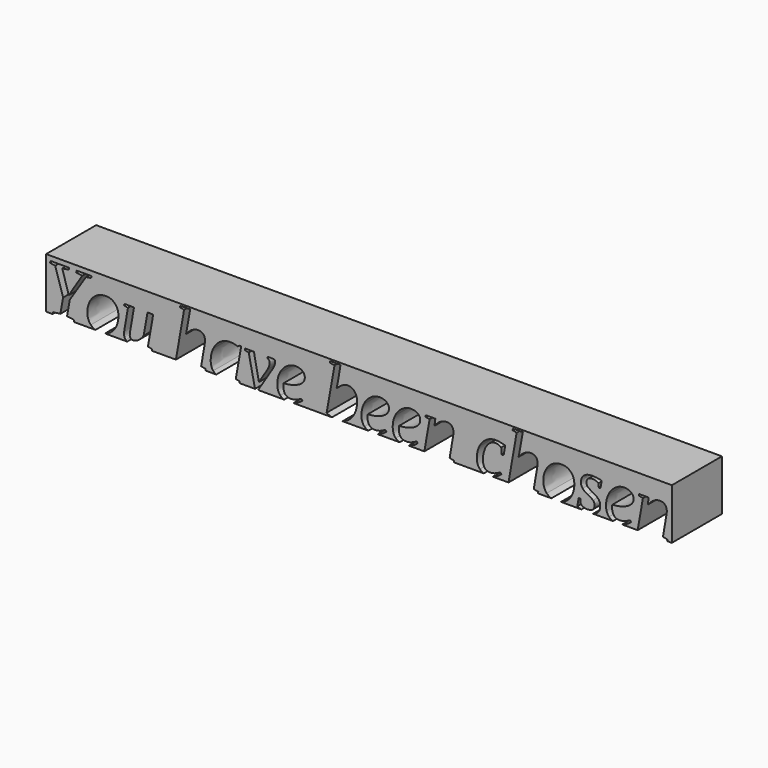
from build123d import *

# Parameters (mm, degrees)
F1_DEPTH = 6.35


with BuildPart() as f1:
    # F0 (on Front) → F1 (new body)
    with BuildSketch(Plane.XZ):
        with BuildLine():
            Line((-250.0064443607, 5.1488298434), (-313.5064443607, 5.1488298434))
            Line((-313.5064443607, 5.1488298434), (-313.5064443607, 0))
            Line((-313.5064443607, 0), (-312.8460801164, 0))
            Line((-312.8460801164, 0), (-312.8114417212, 0.1854830195))
            Line((-312.8114417212, 0.1854830195), (-312.0538664969, 0.2793418969))
            Line((-312.0538664969, 0.2793418969), (-311.7812288055, 1.8224265353))
            Line((-311.7812288055, 1.8224265353), (-312.584616101, 4.4068977653))
            Line((-312.584616101, 4.4068977653), (-313.0974878236, 4.4974045399))
            Line((-313.0974878236, 4.4974045399), (-313.0628494284, 4.6828875594))
            Line((-313.0628494284, 4.6828875594), (-311.1532682213, 4.6828875594))
            Line((-311.1532682213, 4.6828875594), (-311.1879066165, 4.4974045399))
            Line((-311.1879066165, 4.4974045399), (-311.8650313746, 4.4068977653))
            Line((-311.8650313746, 4.4068977653), (-311.2091366007, 2.2168572937))
            Line((-311.2091366007, 2.2168572937), (-309.8370092032, 4.4068977653))
            Line((-309.8370092032, 4.4068977653), (-310.4515613763, 4.4974045399))
            Line((-310.4515613763, 4.4974045399), (-310.4158056135, 4.6828875594))
            Line((-310.4158056135, 4.6828875594), (-308.8939509593, 4.6828875594))
            Line((-308.8939509593, 4.6828875594), (-308.9285893545, 4.4974045399))
            Line((-308.9285893545, 4.4974045399), (-309.4559868558, 4.4068977653))
            Line((-309.4559868558, 4.4068977653), (-311.1041040475, 1.8436565194))
            Line((-311.1041040475, 1.8436565194), (-311.3800938416, 0.2793418969))
            Line((-311.3800938416, 0.2793418969), (-310.6504528069, 0.1854830195))
            Line((-310.6504528069, 0.1854830195), (-310.6850912021, 0))
            Line((-310.6850912021, 0), (-308.4992285411, 0))
            add(Edge.make_bspline(
                [(-308.4992285411, 0), (-308.7698389481, 0.0914468075), (-308.9671385363, 0.3016892486)],
                knots=[0.4349588362, 0.4349588362, 0.4349588362, 1, 1, 1], degree=2))
            add(Edge.make_bspline(
                [(-308.9671385363, 0.3016892486), (-309.3163159074, 0.6737726553), (-309.3163159074, 1.3062027098)],
                knots=[0, 0, 0, 1, 1, 1], degree=2))
            add(Edge.make_bspline(
                [(-309.3163159074, 1.3062027098), (-309.3163159074, 1.8682386064), (-309.0755231923, 2.3464719338)],
                knots=[0, 0, 0, 1, 1, 1], degree=2))
            add(Edge.make_bspline(
                [(-309.0755231923, 2.3464719338), (-308.8347304772, 2.8247052613), (-308.4067786911, 3.0973429527)],
                knots=[0, 0, 0, 1, 1, 1], degree=2))
            add(Edge.make_bspline(
                [(-308.4067786911, 3.0973429527), (-307.9788269051, 3.369980644), (-307.4447251983, 3.369980644)],
                knots=[0, 0, 0, 1, 1, 1], degree=2))
            add(Edge.make_bspline(
                [(-307.4447251983, 3.369980644), (-306.8659287879, 3.369980644), (-306.5167514168, 2.9978972374)],
                knots=[0, 0, 0, 1, 1, 1], degree=2))
            add(Edge.make_bspline(
                [(-306.5167514168, 2.9978972374), (-306.1675740457, 2.6258138307), (-306.1675740457, 1.9933837762)],
                knots=[0, 0, 0, 1, 1, 1], degree=2))
            add(Edge.make_bspline(
                [(-306.1675740457, 1.9933837762), (-306.1675740457, 1.4313478796), (-306.4083667608, 0.9531145522)],
                knots=[0, 0, 0, 1, 1, 1], degree=2))
            add(Edge.make_bspline(
                [(-306.4083667608, 0.9531145522), (-306.6491594759, 0.4748812247), (-307.0765525782, 0.2022435333)],
                knots=[0, 0, 0, 1, 1, 1], degree=2))
            add(Edge.make_bspline(
                [(-307.0765525782, 0.2022435333), (-307.2867741608, 0.0681413996), (-307.523082673, 0)],
                knots=[0, 0, 0, 0.4918693856, 0.4918693856, 0.4918693856], degree=2))
            Line((-307.523082673, 0), (-305.2797553892, 0))
            add(Edge.make_bspline(
                [(-305.2797553892, 0), (-305.3594784168, 0.0425514012), (-305.4194964458, 0.1067086046)],
                knots=[0.6632365324, 0.6632365324, 0.6632365324, 1, 1, 1], degree=2))
            add(Edge.make_bspline(
                [(-305.4194964458, 0.1067086046), (-305.5977165761, 0.2972197783), (-305.5977165761, 0.6525426711)],
                knots=[0, 0, 0, 1, 1, 1], degree=2))
            add(Edge.make_bspline(
                [(-305.5977165761, 0.6525426711), (-305.5977165761, 0.7050589477), (-305.5787213271, 0.839701742)],
                knots=[0, 0, 0, 1, 1, 1], degree=2))
            add(Edge.make_bspline(
                [(-305.5787213271, 0.839701742), (-305.5597260781, 0.9743445363), (-305.2032858177, 3.0414745733)],
                knots=[0, 0, 0, 1, 1, 1], degree=2))
            Line((-305.2032858177, 3.0414745733), (-305.5910123705, 3.1252771424))
            Line((-305.5910123705, 3.1252771424), (-305.5630781808, 3.2828259722))
            Line((-305.5630781808, 3.2828259722), (-304.582029439, 3.2828259722))
            Line((-304.582029439, 3.2828259722), (-304.9384696994, 1.2536864332))
            add(Edge.make_bspline(
                [(-304.9384696994, 1.2536864332), (-305.0178027981, 0.8134436037), (-305.0178027981, 0.6737726553)],
                knots=[0, 0, 0, 1, 1, 1], degree=2))
            add(Edge.make_bspline(
                [(-305.0178027981, 0.6737726553), (-305.0178027981, 0.517341193), (-304.9340002291, 0.4195715291)],
                knots=[0, 0, 0, 1, 1, 1], degree=2))
            add(Edge.make_bspline(
                [(-304.9340002291, 0.4195715291), (-304.85019766, 0.3218018652), (-304.6691841108, 0.3218018652)],
                knots=[0, 0, 0, 1, 1, 1], degree=2))
            add(Edge.make_bspline(
                [(-304.6691841108, 0.3218018652), (-304.4077200953, 0.3218018652), (-304.1037961115, 0.5396885448)],
                knots=[0, 0, 0, 1, 1, 1], degree=2))
            add(Edge.make_bspline(
                [(-304.1037961115, 0.5396885448), (-303.7998721277, 0.7575752244), (-303.6043327999, 1.0760249868)],
                knots=[0, 0, 0, 1, 1, 1], degree=2))
            Line((-303.6043327999, 1.0760249868), (-303.216606247, 3.2828259722))
            Line((-303.216606247, 3.2828259722), (-302.6366924691, 3.2828259722))
            Line((-302.6366924691, 3.2828259722), (-303.1707941759, 0.2447035017))
            Line((-303.1707941759, 0.2447035017), (-302.7596029037, 0.1575488298))
            Line((-302.7596029037, 0.1575488298), (-302.7875370934, 0))
            Line((-302.7875370934, 0), (-300.3326805036, 0))
            Line((-300.3326805036, 0), (-299.5047111212, 4.7208780574))
            Line((-299.5047111212, 4.7208780574), (-299.917019761, 4.8046806264))
            Line((-299.917019761, 4.8046806264), (-299.8890855713, 4.9622294563))
            Line((-299.8890855713, 4.9622294563), (-298.8834547425, 4.9622294563))
            Line((-298.8834547425, 4.9622294563), (-299.253303414, 2.8805736407))
            Line((-299.253303414, 2.8805736407), (-299.3091717934, 2.6157575224))
            add(Edge.make_bspline(
                [(-299.3091717934, 2.6157575224), (-299.0298298965, 2.9822540911), (-298.7102627664, 3.1761173676)],
                knots=[0, 0, 0, 1, 1, 1], degree=2))
            add(Edge.make_bspline(
                [(-298.7102627664, 3.1761173676), (-298.3906956364, 3.369980644), (-298.0834195498, 3.369980644)],
                knots=[0, 0, 0, 1, 1, 1], degree=2))
            add(Edge.make_bspline(
                [(-298.0834195498, 3.369980644), (-297.7314487598, 3.369980644), (-297.5532286295, 3.1794694704)],
                knots=[0, 0, 0, 1, 1, 1], degree=2))
            add(Edge.make_bspline(
                [(-297.5532286295, 3.1794694704), (-297.3750084993, 2.9889582967), (-297.3750084993, 2.6325180362)],
                knots=[0, 0, 0, 1, 1, 1], degree=2))
            add(Edge.make_bspline(
                [(-297.3750084993, 2.6325180362), (-297.3750084993, 2.58447123), (-297.3889755942, 2.4827907795)],
                knots=[0, 0, 0, 1, 1, 1], degree=2))
            add(Edge.make_bspline(
                [(-297.3889755942, 2.4827907795), (-297.402942689, 2.3811103291), (-297.7694392577, 0.2413513989)],
                knots=[0, 0, 0, 1, 1, 1], degree=2))
            Line((-297.7694392577, 0.2413513989), (-297.3124359144, 0.1575488298))
            Line((-297.3124359144, 0.1575488298), (-297.3403701041, 0))
            Line((-297.3403701041, 0), (-296.2384625881, 0))
            add(Edge.make_bspline(
                [(-296.2384625881, 0), (-296.4137627106, 0.0777425781), (-296.5453630656, 0.2374406124)],
                knots=[0.4868098623, 0.4868098623, 0.4868098623, 1, 1, 1], degree=2))
            add(Edge.make_bspline(
                [(-296.5453630656, 0.2374406124), (-296.8017989269, 0.5486274855), (-296.8017989269, 1.0927855006)],
                knots=[0, 0, 0, 1, 1, 1], degree=2))
            add(Edge.make_bspline(
                [(-296.8017989269, 1.0927855006), (-296.8017989269, 1.703985571), (-296.5347480735, 2.2364112265)],
                knots=[0, 0, 0, 1, 1, 1], degree=2))
            add(Edge.make_bspline(
                [(-296.5347480735, 2.2364112265), (-296.2676972201, 2.7688368819), (-295.8207501851, 3.0677327116)],
                knots=[0, 0, 0, 1, 1, 1], degree=2))
            add(Edge.make_bspline(
                [(-295.8207501851, 3.0677327116), (-295.37380315, 3.3666285413), (-294.8497577515, 3.3666285413)],
                knots=[0, 0, 0, 1, 1, 1], degree=2))
            add(Edge.make_bspline(
                [(-294.8497577515, 3.3666285413), (-294.4273928034, 3.3666285413), (-294.0541920292, 3.2191360197)],
                knots=[0, 0, 0, 1, 1, 1], degree=2))
            Line((-294.0541920292, 3.2191360197), (-293.8966431993, 3.3386943516))
            Line((-293.8966431993, 3.3386943516), (-293.7089254446, 3.3386943516))
            Line((-293.7089254446, 3.3386943516), (-294.2597876653, 0.2447035017))
            Line((-294.2597876653, 0.2447035017), (-293.8653569069, 0.1575488298))
            Line((-293.8653569069, 0.1575488298), (-293.8932910966, 0))
            Line((-293.8932910966, 0), (-292.3025629003, 0))
            Line((-292.3025629003, 0), (-292.9468807499, 3.0381224705))
            Line((-292.9468807499, 3.0381224705), (-293.3413115083, 3.1252771424))
            Line((-293.3413115083, 3.1252771424), (-293.3100252159, 3.2828259722))
            Line((-293.3100252159, 3.2828259722), (-292.4161311458, 3.2828259722))
            Line((-292.4161311458, 3.2828259722), (-291.9099636287, 0.7262889319))
            Line((-291.9099636287, 0.7262889319), (-291.0406516456, 2.1442284005))
            add(Edge.make_bspline(
                [(-291.0406516456, 2.1442284005), (-290.8171781281, 2.5073728664), (-290.8171781281, 2.8180010558)],
                knots=[0, 0, 0, 1, 1, 1], degree=2))
            add(Edge.make_bspline(
                [(-290.8171781281, 2.8180010558), (-290.8171781281, 2.9476156959), (-290.890365705, 3.0241553757)],
                knots=[0, 0, 0, 1, 1, 1], degree=2))
            add(Edge.make_bspline(
                [(-290.890365705, 3.0241553757), (-290.963553282, 3.1006950554), (-291.0473558511, 3.1252771424)],
                knots=[0, 0, 0, 1, 1, 1], degree=2))
            Line((-291.0473558511, 3.1252771424), (-291.0194216614, 3.2828259722))
            Line((-291.0194216614, 3.2828259722), (-290.356822682, 3.2828259722))
            add(Edge.make_bspline(
                [(-290.356822682, 3.2828259722), (-290.2651985398, 3.2023755059), (-290.2651985398, 3.0627045575)],
                knots=[0, 0, 0, 1, 1, 1], degree=2))
            add(Edge.make_bspline(
                [(-290.2651985398, 3.0627045575), (-290.2651985398, 2.7554284709), (-290.5557141126, 2.2939556572)],
                knots=[0, 0, 0, 1, 1, 1], degree=2))
            Line((-290.5557141126, 2.2939556572), (-291.9888943483, 0))
            Line((-291.9888943483, 0), (-289.3441800038, 0))
            add(Edge.make_bspline(
                [(-289.3441800038, 0), (-289.5780654992, 0.0788026603), (-289.7394770899, 0.2458208693)],
                knots=[0.4718207721, 0.4718207721, 0.4718207721, 1, 1, 1], degree=2))
            add(Edge.make_bspline(
                [(-289.7394770899, 0.2458208693), (-290.0450771251, 0.5620358965), (-290.0450771251, 1.1520059828)],
                knots=[0, 0, 0, 1, 1, 1], degree=2))
            add(Edge.make_bspline(
                [(-290.0450771251, 1.1520059828), (-290.0450771251, 1.7352718635), (-289.798697572, 2.2397633292)],
                knots=[0, 0, 0, 1, 1, 1], degree=2))
            add(Edge.make_bspline(
                [(-289.798697572, 2.2397633292), (-289.552318019, 2.744254795), (-289.115985976, 3.0571177195)],
                knots=[0, 0, 0, 1, 1, 1], degree=2))
            add(Edge.make_bspline(
                [(-289.115985976, 3.0571177195), (-288.6796539331, 3.369980644), (-288.2014206056, 3.369980644)],
                knots=[0, 0, 0, 1, 1, 1], degree=2))
            add(Edge.make_bspline(
                [(-288.2014206056, 3.369980644), (-287.772351452, 3.369980644), (-287.5120048041, 3.1727652648)],
                knots=[0, 0, 0, 1, 1, 1], degree=2))
            add(Edge.make_bspline(
                [(-287.5120048041, 3.1727652648), (-287.2516581562, 2.9755498856), (-287.2516581562, 2.6537480204)],
                knots=[0, 0, 0, 1, 1, 1], degree=2))
            add(Edge.make_bspline(
                [(-287.2516581562, 2.6537480204), (-287.2516581562, 2.1788667957), (-287.8382761397, 1.8436565194)],
                knots=[0, 0, 0, 1, 1, 1], degree=2))
            add(Edge.make_bspline(
                [(-287.8382761397, 1.8436565194), (-288.4248941231, 1.5084462432), (-289.4126470705, 1.4425215555)],
                knots=[0, 0, 0, 1, 1, 1], degree=2))
            Line((-289.4126470705, 1.4425215555), (-289.4271728492, 1.1877617456))
            add(Edge.make_bspline(
                [(-289.4271728492, 1.1877617456), (-289.4271728492, 0.7441668133), (-289.240572462, 0.5190172444)],
                knots=[0, 0, 0, 1, 1, 1], degree=2))
            add(Edge.make_bspline(
                [(-289.240572462, 0.5190172444), (-289.0539720749, 0.2938676755), (-288.6863581386, 0.2938676755)],
                knots=[0, 0, 0, 1, 1, 1], degree=2))
            add(Edge.make_bspline(
                [(-288.6863581386, 0.2938676755), (-288.3723778465, 0.2938676755), (-288.1070030445, 0.4000175963)],
                knots=[0, 0, 0, 1, 1, 1], degree=2))
            add(Edge.make_bspline(
                [(-288.1070030445, 0.4000175963), (-287.8416282424, 0.5061675172), (-287.6114505194, 0.6424863628)],
                knots=[0, 0, 0, 1, 1, 1], degree=2))
            Line((-287.6114505194, 0.6424863628), (-287.5097700689, 0.4961112089))
            add(Edge.make_bspline(
                [(-287.5097700689, 0.4961112089), (-287.8315719341, 0.2234735175), (-288.1891295622, 0.0765396797)],
                knots=[0, 0, 0, 1, 1, 1], degree=2))
            add(Edge.make_bspline(
                [(-288.1891295622, 0.0765396797), (-288.2991995892, 0.031307778), (-288.4058812363, 0)],
                knots=[0, 0, 0, 0.3078385647, 0.3078385647, 0.3078385647], degree=2))
            Line((-288.4058812363, 0), (-284.4901280472, 0))
            add(Edge.make_bspline(
                [(-284.4901280472, 0), (-284.5063254791, 0.0040723352), (-284.5224878236, 0.0083802569)],
                knots=[0.9453131869, 0.9453131869, 0.9453131869, 1, 1, 1], degree=2))
            add(Edge.make_bspline(
                [(-284.5224878236, 0.0083802569), (-284.8180315505, 0.0871546718), (-285.0370355977, 0.2234735175)],
                knots=[0, 0, 0, 1, 1, 1], degree=2))
            Line((-285.0370355977, 0.2234735175), (-284.2381177726, 4.7208780574))
            Line((-284.2381177726, 4.7208780574), (-284.7018253214, 4.8046806264))
            Line((-284.7018253214, 4.8046806264), (-284.6738911317, 4.9622294563))
            Line((-284.6738911317, 4.9622294563), (-283.6269177022, 4.9622294563))
            Line((-283.6269177022, 4.9622294563), (-283.8850296149, 3.4224969206))
            add(Edge.make_bspline(
                [(-283.8850296149, 3.4224969206), (-283.9442500971, 3.0235966919), (-284.0213484606, 2.7476068978)],
                knots=[0, 0, 0, 1, 1, 1], degree=2))
            add(Edge.make_bspline(
                [(-284.0213484606, 2.7476068978), (-283.7420065637, 3.0347703678), (-283.4470215206, 3.2023755059)],
                knots=[0, 0, 0, 1, 1, 1], degree=2))
            add(Edge.make_bspline(
                [(-283.4470215206, 3.2023755059), (-283.1520364775, 3.369980644), (-282.9039808731, 3.369980644)],
                knots=[0, 0, 0, 1, 1, 1], degree=2))
            add(Edge.make_bspline(
                [(-282.9039808731, 3.369980644), (-282.4670901464, 3.369980644), (-282.2056261309, 3.0571177195)],
                knots=[0, 0, 0, 1, 1, 1], degree=2))
            add(Edge.make_bspline(
                [(-282.2056261309, 3.0571177195), (-281.9441621154, 2.744254795), (-281.9441621154, 2.2034488826)],
                knots=[0, 0, 0, 1, 1, 1], degree=2))
            add(Edge.make_bspline(
                [(-281.9441621154, 2.2034488826), (-281.9441621154, 1.6023051205), (-282.2039500795, 1.0698794651)],
                knots=[0, 0, 0, 1, 1, 1], degree=2))
            add(Edge.make_bspline(
                [(-282.2039500795, 1.0698794651), (-282.4637380436, 0.5374538096), (-282.9213000707, 0.2335298258)],
                knots=[0, 0, 0, 1, 1, 1], degree=2))
            add(Edge.make_bspline(
                [(-282.9213000707, 0.2335298258), (-283.158652726, 0.075874338), (-283.4184049976, 0)],
                knots=[0, 0, 0, 0.5187332891, 0.5187332891, 0.5187332891], degree=2))
            Line((-283.4184049976, 0), (-280.8063742674, 0))
            add(Edge.make_bspline(
                [(-280.8063742674, 0), (-281.0402597628, 0.0788026603), (-281.2016713535, 0.2458208693)],
                knots=[0.4718207721, 0.4718207721, 0.4718207721, 1, 1, 1], degree=2))
            add(Edge.make_bspline(
                [(-281.2016713535, 0.2458208693), (-281.5072713887, 0.5620358965), (-281.5072713887, 1.1520059828)],
                knots=[0, 0, 0, 1, 1, 1], degree=2))
            add(Edge.make_bspline(
                [(-281.5072713887, 1.1520059828), (-281.5072713887, 1.7352718635), (-281.2608918356, 2.2397633292)],
                knots=[0, 0, 0, 1, 1, 1], degree=2))
            add(Edge.make_bspline(
                [(-281.2608918356, 2.2397633292), (-281.0145122825, 2.744254795), (-280.5781802396, 3.0571177195)],
                knots=[0, 0, 0, 1, 1, 1], degree=2))
            add(Edge.make_bspline(
                [(-280.5781802396, 3.0571177195), (-280.1418481967, 3.369980644), (-279.6636148692, 3.369980644)],
                knots=[0, 0, 0, 1, 1, 1], degree=2))
            add(Edge.make_bspline(
                [(-279.6636148692, 3.369980644), (-279.2345457156, 3.369980644), (-278.9741990677, 3.1727652648)],
                knots=[0, 0, 0, 1, 1, 1], degree=2))
            add(Edge.make_bspline(
                [(-278.9741990677, 3.1727652648), (-278.7138524198, 2.9755498856), (-278.7138524198, 2.6537480204)],
                knots=[0, 0, 0, 1, 1, 1], degree=2))
            add(Edge.make_bspline(
                [(-278.7138524198, 2.6537480204), (-278.7138524198, 2.1788667957), (-279.3004704033, 1.8436565194)],
                knots=[0, 0, 0, 1, 1, 1], degree=2))
            add(Edge.make_bspline(
                [(-279.3004704033, 1.8436565194), (-279.8870883867, 1.5084462432), (-280.8748413341, 1.4425215555)],
                knots=[0, 0, 0, 1, 1, 1], degree=2))
            Line((-280.8748413341, 1.4425215555), (-280.8893671127, 1.1877617456))
            add(Edge.make_bspline(
                [(-280.8893671127, 1.1877617456), (-280.8893671127, 0.7441668133), (-280.7027667256, 0.5190172444)],
                knots=[0, 0, 0, 1, 1, 1], degree=2))
            add(Edge.make_bspline(
                [(-280.7027667256, 0.5190172444), (-280.5161663385, 0.2938676755), (-280.1485524022, 0.2938676755)],
                knots=[0, 0, 0, 1, 1, 1], degree=2))
            add(Edge.make_bspline(
                [(-280.1485524022, 0.2938676755), (-279.8345721101, 0.2938676755), (-279.5691973081, 0.4000175963)],
                knots=[0, 0, 0, 1, 1, 1], degree=2))
            add(Edge.make_bspline(
                [(-279.5691973081, 0.4000175963), (-279.303822506, 0.5061675172), (-279.073644783, 0.6424863628)],
                knots=[0, 0, 0, 1, 1, 1], degree=2))
            Line((-279.073644783, 0.6424863628), (-278.9719643325, 0.4961112089))
            add(Edge.make_bspline(
                [(-278.9719643325, 0.4961112089), (-279.2937661977, 0.2234735175), (-279.6513238257, 0.0765396797)],
                knots=[0, 0, 0, 1, 1, 1], degree=2))
            add(Edge.make_bspline(
                [(-279.6513238257, 0.0765396797), (-279.7613938528, 0.031307778), (-279.8680754999, 0)],
                knots=[0, 0, 0, 0.3078385647, 0.3078385647, 0.3078385647], degree=2))
            Line((-279.8680754999, 0), (-277.6319329512, 0))
            add(Edge.make_bspline(
                [(-277.6319329512, 0), (-277.8658184466, 0.0788026603), (-278.0272300373, 0.2458208693)],
                knots=[0.4718207721, 0.4718207721, 0.4718207721, 1, 1, 1], degree=2))
            add(Edge.make_bspline(
                [(-278.0272300373, 0.2458208693), (-278.3328300724, 0.5620358965), (-278.3328300724, 1.1520059828)],
                knots=[0, 0, 0, 1, 1, 1], degree=2))
            add(Edge.make_bspline(
                [(-278.3328300724, 1.1520059828), (-278.3328300724, 1.7352718635), (-278.0864505194, 2.2397633292)],
                knots=[0, 0, 0, 1, 1, 1], degree=2))
            add(Edge.make_bspline(
                [(-278.0864505194, 2.2397633292), (-277.8400709663, 2.744254795), (-277.4037389234, 3.0571177195)],
                knots=[0, 0, 0, 1, 1, 1], degree=2))
            add(Edge.make_bspline(
                [(-277.4037389234, 3.0571177195), (-276.9674068805, 3.369980644), (-276.489173553, 3.369980644)],
                knots=[0, 0, 0, 1, 1, 1], degree=2))
            add(Edge.make_bspline(
                [(-276.489173553, 3.369980644), (-276.0601043994, 3.369980644), (-275.7997577515, 3.1727652648)],
                knots=[0, 0, 0, 1, 1, 1], degree=2))
            add(Edge.make_bspline(
                [(-275.7997577515, 3.1727652648), (-275.5394111036, 2.9755498856), (-275.5394111036, 2.6537480204)],
                knots=[0, 0, 0, 1, 1, 1], degree=2))
            add(Edge.make_bspline(
                [(-275.5394111036, 2.6537480204), (-275.5394111036, 2.1788667957), (-276.1260290871, 1.8436565194)],
                knots=[0, 0, 0, 1, 1, 1], degree=2))
            add(Edge.make_bspline(
                [(-276.1260290871, 1.8436565194), (-276.7126470705, 1.5084462432), (-277.7004000179, 1.4425215555)],
                knots=[0, 0, 0, 1, 1, 1], degree=2))
            Line((-277.7004000179, 1.4425215555), (-277.7149257965, 1.1877617456))
            add(Edge.make_bspline(
                [(-277.7149257965, 1.1877617456), (-277.7149257965, 0.7441668133), (-277.5283254094, 0.5190172444)],
                knots=[0, 0, 0, 1, 1, 1], degree=2))
            add(Edge.make_bspline(
                [(-277.5283254094, 0.5190172444), (-277.3417250223, 0.2938676755), (-276.974111086, 0.2938676755)],
                knots=[0, 0, 0, 1, 1, 1], degree=2))
            add(Edge.make_bspline(
                [(-276.974111086, 0.2938676755), (-276.6601307939, 0.2938676755), (-276.3947559919, 0.4000175963)],
                knots=[0, 0, 0, 1, 1, 1], degree=2))
            add(Edge.make_bspline(
                [(-276.3947559919, 0.4000175963), (-276.1293811898, 0.5061675172), (-275.8992034668, 0.6424863628)],
                knots=[0, 0, 0, 1, 1, 1], degree=2))
            Line((-275.8992034668, 0.6424863628), (-275.7975230163, 0.4961112089))
            add(Edge.make_bspline(
                [(-275.7975230163, 0.4961112089), (-276.1193248815, 0.2234735175), (-276.4768825095, 0.0765396797)],
                knots=[0, 0, 0, 1, 1, 1], degree=2))
            add(Edge.make_bspline(
                [(-276.4768825095, 0.0765396797), (-276.5869525366, 0.031307778), (-276.6936341837, 0)],
                knots=[0, 0, 0, 0.3078385647, 0.3078385647, 0.3078385647], degree=2))
            Line((-276.6936341837, 0), (-275.123750361, 0))
            Line((-275.123750361, 0), (-274.5896486542, 3.0414745733))
            Line((-274.5896486542, 3.0414745733), (-275.0008399264, 3.1286292451))
            Line((-275.0008399264, 3.1286292451), (-274.9729057367, 3.286178075))
            Line((-274.9729057367, 3.286178075), (-274.0030306707, 3.286178075))
            Line((-274.0030306707, 3.286178075), (-274.0968895481, 2.6157575224))
            add(Edge.make_bspline(
                [(-274.0968895481, 2.6157575224), (-273.8041392401, 2.9923103994), (-273.4896002642, 3.1811455217)],
                knots=[0, 0, 0, 1, 1, 1], degree=2))
            add(Edge.make_bspline(
                [(-273.4896002642, 3.1811455217), (-273.1750612884, 3.369980644), (-272.8711373045, 3.369980644)],
                knots=[0, 0, 0, 1, 1, 1], degree=2))
            add(Edge.make_bspline(
                [(-272.8711373045, 3.369980644), (-272.5191665145, 3.369980644), (-272.3409463843, 3.1794694704)],
                knots=[0, 0, 0, 1, 1, 1], degree=2))
            add(Edge.make_bspline(
                [(-272.3409463843, 3.1794694704), (-272.162726254, 2.9889582967), (-272.162726254, 2.6325180362)],
                knots=[0, 0, 0, 1, 1, 1], degree=2))
            add(Edge.make_bspline(
                [(-272.162726254, 2.6325180362), (-272.162726254, 2.58447123), (-272.1766933489, 2.4827907795)],
                knots=[0, 0, 0, 1, 1, 1], degree=2))
            add(Edge.make_bspline(
                [(-272.1766933489, 2.4827907795), (-272.1906604437, 2.3811103291), (-272.5571570124, 0.2413513989)],
                knots=[0, 0, 0, 1, 1, 1], degree=2))
            Line((-272.5571570124, 0.2413513989), (-272.1001536691, 0.1575488298))
            Line((-272.1001536691, 0.1575488298), (-272.1280878588, 0))
            Line((-272.1280878588, 0), (-269.0863015193, 0))
            add(Edge.make_bspline(
                [(-269.0863015193, 0), (-269.3234446734, 0.0808967531), (-269.4877482495, 0.25475981)],
                knots=[0.4652900658, 0.4652900658, 0.4652900658, 1, 1, 1], degree=2))
            add(Edge.make_bspline(
                [(-269.4877482495, 0.25475981), (-269.795024336, 0.5799137779), (-269.795024336, 1.1520059828)],
                knots=[0, 0, 0, 1, 1, 1], degree=2))
            add(Edge.make_bspline(
                [(-269.795024336, 1.1520059828), (-269.795024336, 1.7598539504), (-269.5508795182, 2.2609933134)],
                knots=[0, 0, 0, 1, 1, 1], degree=2))
            add(Edge.make_bspline(
                [(-269.5508795182, 2.2609933134), (-269.3067347003, 2.7621326764), (-268.8542008273, 3.0660566602)],
                knots=[0, 0, 0, 1, 1, 1], degree=2))
            add(Edge.make_bspline(
                [(-268.8542008273, 3.0660566602), (-268.4016669544, 3.369980644), (-267.9055557455, 3.369980644)],
                knots=[0, 0, 0, 1, 1, 1], degree=2))
            add(Edge.make_bspline(
                [(-267.9055557455, 3.369980644), (-267.6586175087, 3.369980644), (-267.3792756118, 3.3174643674)],
                knots=[0, 0, 0, 1, 1, 1], degree=2))
            add(Edge.make_bspline(
                [(-267.3792756118, 3.3174643674), (-267.0999337149, 3.2649480908), (-266.9178027981, 3.1878497273)],
                knots=[0, 0, 0, 1, 1, 1], degree=2))
            Line((-266.9178027981, 3.1878497273), (-267.075351628, 2.2727256731))
            Line((-267.075351628, 2.2727256731), (-267.267538853, 2.2727256731))
            Line((-267.267538853, 2.2727256731), (-267.3234072324, 2.8805736407))
            add(Edge.make_bspline(
                [(-267.3234072324, 2.8805736407), (-267.5424112796, 3.1006950554), (-267.9100252159, 3.1006950554)],
                knots=[0, 0, 0, 1, 1, 1], degree=2))
            add(Edge.make_bspline(
                [(-267.9100252159, 3.1006950554), (-268.2452354921, 3.1006950554), (-268.5363097487, 2.852639451)],
                knots=[0, 0, 0, 1, 1, 1], degree=2))
            add(Edge.make_bspline(
                [(-268.5363097487, 2.852639451), (-268.8273840052, 2.6045838466), (-269.0022520327, 2.1615475981)],
                knots=[0, 0, 0, 1, 1, 1], degree=2))
            add(Edge.make_bspline(
                [(-269.0022520327, 2.1615475981), (-269.1771200601, 1.7185113496), (-269.1771200601, 1.1877617456)],
                knots=[0, 0, 0, 1, 1, 1], degree=2))
            add(Edge.make_bspline(
                [(-269.1771200601, 1.1877617456), (-269.1771200601, 0.2938676755), (-268.4575353338, 0.2938676755)],
                knots=[0, 0, 0, 1, 1, 1], degree=2))
            add(Edge.make_bspline(
                [(-268.4575353338, 0.2938676755), (-267.9580720221, 0.2938676755), (-267.4172661098, 0.6424863628)],
                knots=[0, 0, 0, 1, 1, 1], degree=2))
            Line((-267.4172661098, 0.6424863628), (-267.3122335565, 0.4961112089))
            add(Edge.make_bspline(
                [(-267.3122335565, 0.4961112089), (-267.5949275562, 0.2335298258), (-267.9480157138, 0.0815678339)],
                knots=[0, 0, 0, 1, 1, 1], degree=2))
            add(Edge.make_bspline(
                [(-267.9480157138, 0.0815678339), (-268.06078716, 0.0330332874), (-268.1699112512, 0)],
                knots=[0, 0, 0, 0.3193860903, 0.3193860903, 0.3193860903], degree=2))
            Line((-268.1699112512, 0), (-266.5825925219, 0))
            Line((-266.5825925219, 0), (-265.7546231395, 4.7208780574))
            Line((-265.7546231395, 4.7208780574), (-266.1669317793, 4.8046806264))
            Line((-266.1669317793, 4.8046806264), (-266.1389975896, 4.9622294563))
            Line((-266.1389975896, 4.9622294563), (-265.1333667608, 4.9622294563))
            Line((-265.1333667608, 4.9622294563), (-265.5032154323, 2.8805736407))
            Line((-265.5032154323, 2.8805736407), (-265.5590838117, 2.6157575224))
            add(Edge.make_bspline(
                [(-265.5590838117, 2.6157575224), (-265.2797419148, 2.9822540911), (-264.9601747847, 3.1761173676)],
                knots=[0, 0, 0, 1, 1, 1], degree=2))
            add(Edge.make_bspline(
                [(-264.9601747847, 3.1761173676), (-264.6406076547, 3.369980644), (-264.3333315681, 3.369980644)],
                knots=[0, 0, 0, 1, 1, 1], degree=2))
            add(Edge.make_bspline(
                [(-264.3333315681, 3.369980644), (-263.9813607781, 3.369980644), (-263.8031406478, 3.1794694704)],
                knots=[0, 0, 0, 1, 1, 1], degree=2))
            add(Edge.make_bspline(
                [(-263.8031406478, 3.1794694704), (-263.6249205176, 2.9889582967), (-263.6249205176, 2.6325180362)],
                knots=[0, 0, 0, 1, 1, 1], degree=2))
            add(Edge.make_bspline(
                [(-263.6249205176, 2.6325180362), (-263.6249205176, 2.58447123), (-263.6388876125, 2.4827907795)],
                knots=[0, 0, 0, 1, 1, 1], degree=2))
            add(Edge.make_bspline(
                [(-263.6388876125, 2.4827907795), (-263.6528547073, 2.3811103291), (-264.019351276, 0.2413513989)],
                knots=[0, 0, 0, 1, 1, 1], degree=2))
            Line((-264.019351276, 0.2413513989), (-263.5623479327, 0.1575488298))
            Line((-263.5623479327, 0.1575488298), (-263.5902821224, 0))
            Line((-263.5902821224, 0), (-262.2346235789, 0))
            add(Edge.make_bspline(
                [(-262.2346235789, 0), (-262.505233986, 0.0914468075), (-262.7025335741, 0.3016892486)],
                knots=[0.4349588362, 0.4349588362, 0.4349588362, 1, 1, 1], degree=2))
            add(Edge.make_bspline(
                [(-262.7025335741, 0.3016892486), (-263.0517109452, 0.6737726553), (-263.0517109452, 1.3062027098)],
                knots=[0, 0, 0, 1, 1, 1], degree=2))
            add(Edge.make_bspline(
                [(-263.0517109452, 1.3062027098), (-263.0517109452, 1.8682386064), (-262.8109182301, 2.3464719338)],
                knots=[0, 0, 0, 1, 1, 1], degree=2))
            add(Edge.make_bspline(
                [(-262.8109182301, 2.3464719338), (-262.570125515, 2.8247052613), (-262.142173729, 3.0973429527)],
                knots=[0, 0, 0, 1, 1, 1], degree=2))
            add(Edge.make_bspline(
                [(-262.142173729, 3.0973429527), (-261.7142219429, 3.369980644), (-261.1801202361, 3.369980644)],
                knots=[0, 0, 0, 1, 1, 1], degree=2))
            add(Edge.make_bspline(
                [(-261.1801202361, 3.369980644), (-260.6013238257, 3.369980644), (-260.2521464546, 2.9978972374)],
                knots=[0, 0, 0, 1, 1, 1], degree=2))
            add(Edge.make_bspline(
                [(-260.2521464546, 2.9978972374), (-259.9029690835, 2.6258138307), (-259.9029690835, 1.9933837762)],
                knots=[0, 0, 0, 1, 1, 1], degree=2))
            add(Edge.make_bspline(
                [(-259.9029690835, 1.9933837762), (-259.9029690835, 1.4313478796), (-260.1437617986, 0.9531145522)],
                knots=[0, 0, 0, 1, 1, 1], degree=2))
            add(Edge.make_bspline(
                [(-260.1437617986, 0.9531145522), (-260.3845545138, 0.4748812247), (-260.811947616, 0.2022435333)],
                knots=[0, 0, 0, 1, 1, 1], degree=2))
            add(Edge.make_bspline(
                [(-260.811947616, 0.2022435333), (-261.0221691986, 0.0681413996), (-261.2584777109, 0)],
                knots=[0, 0, 0, 0.4918693856, 0.4918693856, 0.4918693856], degree=2))
            Line((-261.2584777109, 0), (-259.1782918063, 0))
            add(Edge.make_bspline(
                [(-259.1782918063, 0), (-259.3890007317, 0.0531343537), (-259.6023972025, 0.146375154)],
                knots=[0.5698616218, 0.5698616218, 0.5698616218, 1, 1, 1], degree=2))
            Line((-259.6023972025, 0.146375154), (-259.4593741513, 0.9363540384))
            Line((-259.4593741513, 0.9363540384), (-259.3018253214, 0.9363540384))
            Line((-259.3018253214, 0.9363540384), (-259.2426048393, 0.4570033433))
            add(Edge.make_bspline(
                [(-259.2426048393, 0.4570033433), (-259.1520980647, 0.3597923632), (-258.986168978, 0.2826939996)],
                knots=[0, 0, 0, 1, 1, 1], degree=2))
            add(Edge.make_bspline(
                [(-258.986168978, 0.2826939996), (-258.8202398912, 0.2055956361), (-258.6101747847, 0.2055956361)],
                knots=[0, 0, 0, 1, 1, 1], degree=2))
            add(Edge.make_bspline(
                [(-258.6101747847, 0.2055956361), (-257.8458953549, 0.2055956361), (-257.8458953549, 0.8313214851)],
                knots=[0, 0, 0, 1, 1, 1], degree=2))
            add(Edge.make_bspline(
                [(-257.8458953549, 0.8313214851), (-257.8458953549, 1.0369171212), (-258.0084723389, 1.1978180538)],
                knots=[0, 0, 0, 1, 1, 1], degree=2))
            add(Edge.make_bspline(
                [(-258.0084723389, 1.1978180538), (-258.1710493228, 1.3587189865), (-258.5375458916, 1.5363804329)],
                knots=[0, 0, 0, 1, 1, 1], degree=2))
            add(Edge.make_bspline(
                [(-258.5375458916, 1.5363804329), (-258.8895166816, 1.7073376738), (-259.0610326063, 1.915168045)],
                knots=[0, 0, 0, 1, 1, 1], degree=2))
            add(Edge.make_bspline(
                [(-259.0610326063, 1.915168045), (-259.232548531, 2.1229984163), (-259.232548531, 2.4023403132)],
                knots=[0, 0, 0, 1, 1, 1], degree=2))
            add(Edge.make_bspline(
                [(-259.232548531, 2.4023403132), (-259.232548531, 2.8638131269), (-258.9213616579, 3.1168968854)],
                knots=[0, 0, 0, 1, 1, 1], degree=2))
            add(Edge.make_bspline(
                [(-258.9213616579, 3.1168968854), (-258.6101747847, 3.369980644), (-258.0593125641, 3.369980644)],
                knots=[0, 0, 0, 1, 1, 1], degree=2))
            add(Edge.make_bspline(
                [(-258.0593125641, 3.369980644), (-257.6637644381, 3.369980644), (-257.1229585257, 3.2470702094)],
                knots=[0, 0, 0, 1, 1, 1], degree=2))
            Line((-257.1229585257, 3.2470702094), (-257.2525731659, 2.5174291747))
            Line((-257.2525731659, 2.5174291747), (-257.4168262013, 2.5174291747))
            Line((-257.4168262013, 2.5174291747), (-257.4648730075, 2.8950994193))
            add(Edge.make_bspline(
                [(-257.4648730075, 2.8950994193), (-257.6849944223, 3.0906387471), (-258.0447867855, 3.0906387471)],
                knots=[0, 0, 0, 1, 1, 1], degree=2))
            add(Edge.make_bspline(
                [(-258.0447867855, 3.0906387471), (-258.3308328879, 3.0906387471), (-258.5023488126, 2.9593480556)],
                knots=[0, 0, 0, 1, 1, 1], degree=2))
            add(Edge.make_bspline(
                [(-258.5023488126, 2.9593480556), (-258.6738647372, 2.8280573641), (-258.6738647372, 2.5520675699)],
                knots=[0, 0, 0, 1, 1, 1], degree=2))
            add(Edge.make_bspline(
                [(-258.6738647372, 2.5520675699), (-258.6738647372, 2.3643498152), (-258.5269308995, 2.2207680802)],
                knots=[0, 0, 0, 1, 1, 1], degree=2))
            add(Edge.make_bspline(
                [(-258.5269308995, 2.2207680802), (-258.3799970617, 2.0771863452), (-257.9710405247, 1.8682386064)],
                knots=[0, 0, 0, 1, 1, 1], degree=2))
            add(Edge.make_bspline(
                [(-257.9710405247, 1.8682386064), (-257.6078960587, 1.6794034841), (-257.4402909206, 1.4631928559)],
                knots=[0, 0, 0, 1, 1, 1], degree=2))
            add(Edge.make_bspline(
                [(-257.4402909206, 1.4631928559), (-257.2726857825, 1.2469822277), (-257.2726857825, 0.964288228)],
                knots=[0, 0, 0, 1, 1, 1], degree=2))
            add(Edge.make_bspline(
                [(-257.2726857825, 0.964288228), (-257.2726857825, 0.4368907267), (-257.6078960587, 0.1832482844)],
                knots=[0, 0, 0, 1, 1, 1], degree=2))
            add(Edge.make_bspline(
                [(-257.6078960587, 0.1832482844), (-257.7665128529, 0.0632282434), (-258.0026867274, 0)],
                knots=[0, 0, 0, 0.4731859534, 0.4731859534, 0.4731859534], degree=2))
            Line((-258.0026867274, 0), (-255.9851706777, 0))
            add(Edge.make_bspline(
                [(-255.9851706777, 0), (-256.2190561732, 0.0788026603), (-256.3804677638, 0.2458208693)],
                knots=[0.4718207721, 0.4718207721, 0.4718207721, 1, 1, 1], degree=2))
            add(Edge.make_bspline(
                [(-256.3804677638, 0.2458208693), (-256.686067799, 0.5620358965), (-256.686067799, 1.1520059828)],
                knots=[0, 0, 0, 1, 1, 1], degree=2))
            add(Edge.make_bspline(
                [(-256.686067799, 1.1520059828), (-256.686067799, 1.7352718635), (-256.4396882459, 2.2397633292)],
                knots=[0, 0, 0, 1, 1, 1], degree=2))
            add(Edge.make_bspline(
                [(-256.4396882459, 2.2397633292), (-256.1933086929, 2.744254795), (-255.75697665, 3.0571177195)],
                knots=[0, 0, 0, 1, 1, 1], degree=2))
            add(Edge.make_bspline(
                [(-255.75697665, 3.0571177195), (-255.320644607, 3.369980644), (-254.8424112796, 3.369980644)],
                knots=[0, 0, 0, 1, 1, 1], degree=2))
            add(Edge.make_bspline(
                [(-254.8424112796, 3.369980644), (-254.4133421259, 3.369980644), (-254.152995478, 3.1727652648)],
                knots=[0, 0, 0, 1, 1, 1], degree=2))
            add(Edge.make_bspline(
                [(-254.152995478, 3.1727652648), (-253.8926488301, 2.9755498856), (-253.8926488301, 2.6537480204)],
                knots=[0, 0, 0, 1, 1, 1], degree=2))
            add(Edge.make_bspline(
                [(-253.8926488301, 2.6537480204), (-253.8926488301, 2.1788667957), (-254.4792668136, 1.8436565194)],
                knots=[0, 0, 0, 1, 1, 1], degree=2))
            add(Edge.make_bspline(
                [(-254.4792668136, 1.8436565194), (-255.0658847971, 1.5084462432), (-256.0536377445, 1.4425215555)],
                knots=[0, 0, 0, 1, 1, 1], degree=2))
            Line((-256.0536377445, 1.4425215555), (-256.0681635231, 1.1877617456))
            add(Edge.make_bspline(
                [(-256.0681635231, 1.1877617456), (-256.0681635231, 0.7441668133), (-255.881563136, 0.5190172444)],
                knots=[0, 0, 0, 1, 1, 1], degree=2))
            add(Edge.make_bspline(
                [(-255.881563136, 0.5190172444), (-255.6949627489, 0.2938676755), (-255.3273488126, 0.2938676755)],
                knots=[0, 0, 0, 1, 1, 1], degree=2))
            add(Edge.make_bspline(
                [(-255.3273488126, 0.2938676755), (-255.0133685205, 0.2938676755), (-254.7479937184, 0.4000175963)],
                knots=[0, 0, 0, 1, 1, 1], degree=2))
            add(Edge.make_bspline(
                [(-254.7479937184, 0.4000175963), (-254.4826189164, 0.5061675172), (-254.2524411933, 0.6424863628)],
                knots=[0, 0, 0, 1, 1, 1], degree=2))
            Line((-254.2524411933, 0.6424863628), (-254.1507607429, 0.4961112089))
            add(Edge.make_bspline(
                [(-254.1507607429, 0.4961112089), (-254.4725626081, 0.2234735175), (-254.8301202361, 0.0765396797)],
                knots=[0, 0, 0, 1, 1, 1], degree=2))
            add(Edge.make_bspline(
                [(-254.8301202361, 0.0765396797), (-254.9401902631, 0.031307778), (-255.0468719102, 0)],
                knots=[0, 0, 0, 0.3078385647, 0.3078385647, 0.3078385647], degree=2))
            Line((-255.0468719102, 0), (-253.4769880876, 0))
            Line((-253.4769880876, 0), (-252.9428863807, 3.0414745733))
            Line((-252.9428863807, 3.0414745733), (-253.354077653, 3.1286292451))
            Line((-253.354077653, 3.1286292451), (-253.3261434633, 3.286178075))
            Line((-253.3261434633, 3.286178075), (-252.3562683973, 3.286178075))
            Line((-252.3562683973, 3.286178075), (-252.4501272746, 2.6157575224))
            add(Edge.make_bspline(
                [(-252.4501272746, 2.6157575224), (-252.1573769667, 2.9923103994), (-251.8428379908, 3.1811455217)],
                knots=[0, 0, 0, 1, 1, 1], degree=2))
            add(Edge.make_bspline(
                [(-251.8428379908, 3.1811455217), (-251.5282990149, 3.369980644), (-251.2243750311, 3.369980644)],
                knots=[0, 0, 0, 1, 1, 1], degree=2))
            add(Edge.make_bspline(
                [(-251.2243750311, 3.369980644), (-250.872404241, 3.369980644), (-250.6941841108, 3.1794694704)],
                knots=[0, 0, 0, 1, 1, 1], degree=2))
            add(Edge.make_bspline(
                [(-250.6941841108, 3.1794694704), (-250.5159639806, 2.9889582967), (-250.5159639806, 2.6325180362)],
                knots=[0, 0, 0, 1, 1, 1], degree=2))
            add(Edge.make_bspline(
                [(-250.5159639806, 2.6325180362), (-250.5159639806, 2.58447123), (-250.5299310754, 2.4827907795)],
                knots=[0, 0, 0, 1, 1, 1], degree=2))
            add(Edge.make_bspline(
                [(-250.5299310754, 2.4827907795), (-250.5438981703, 2.3811103291), (-250.910394739, 0.2413513989)],
                knots=[0, 0, 0, 1, 1, 1], degree=2))
            Line((-250.910394739, 0.2413513989), (-250.4533913957, 0.1575488298))
            Line((-250.4533913957, 0.1575488298), (-250.4813255854, 0))
            Line((-250.4813255854, 0), (-250.0064443607, 0))
            Line((-250.0064443607, 0), (-250.0064443607, 5.1488298434))
        make_face()
    extrude(amount=F1_DEPTH)


solid = f1.part
